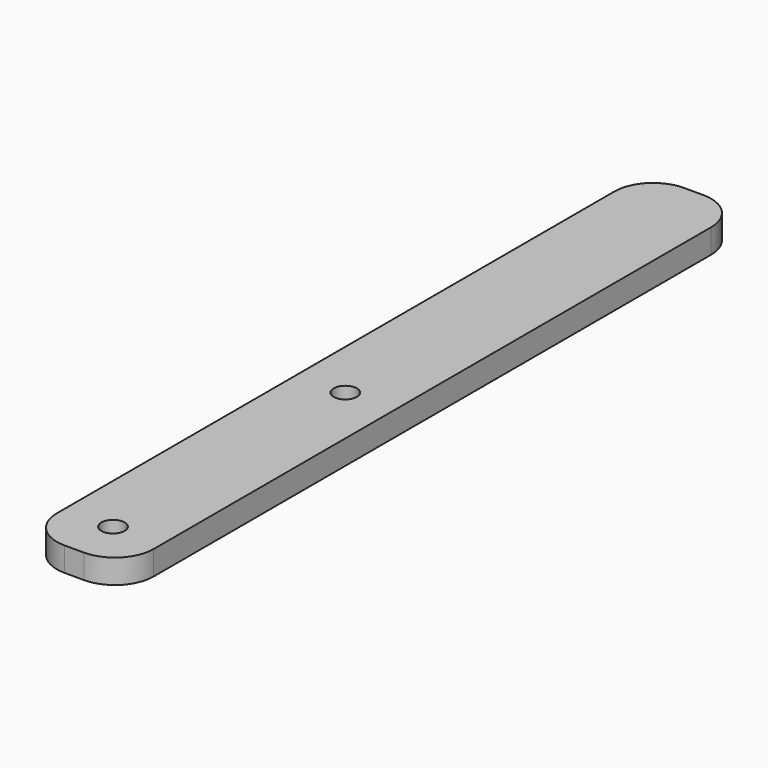
from build123d import *

# Parameters (mm, degrees)
F0_R     = 1.524
F1_DEPTH = 3.175
F2_R     = 5.08


# Not quite as in the source:
# - a feature names something its author has since deleted; it is built from what else it names


with BuildPart() as f1:
    # F0 (on Top) → F1 (new body)
    with BuildSketch(Plane.XY):
        Polygon((-6.35, -25.4), (6.35, -25.4), (6.35, 25.4), (6.35, 76.2), (-6.35, 76.2), (-6.35, 25.4), align=None)
        with Locations((0, -19.05)):
            Circle(F0_R, mode=Mode.SUBTRACT)
        with Locations((0, 19.05)):
            Circle(F0_R, mode=Mode.SUBTRACT)
    extrude(amount=F1_DEPTH)

    # F2
    f2_edges = [f1.edges().sort_by_distance(p)[0] for p in [
        (-6.35, 76.2, 1.5875),
        (6.35, 76.2, 1.5875),
        (-6.35, -25.4, 1.5875),
        (6.35, -25.4, 1.5875),
    ]]
    fillet(f2_edges, radius=F2_R)


solid = f1.part
